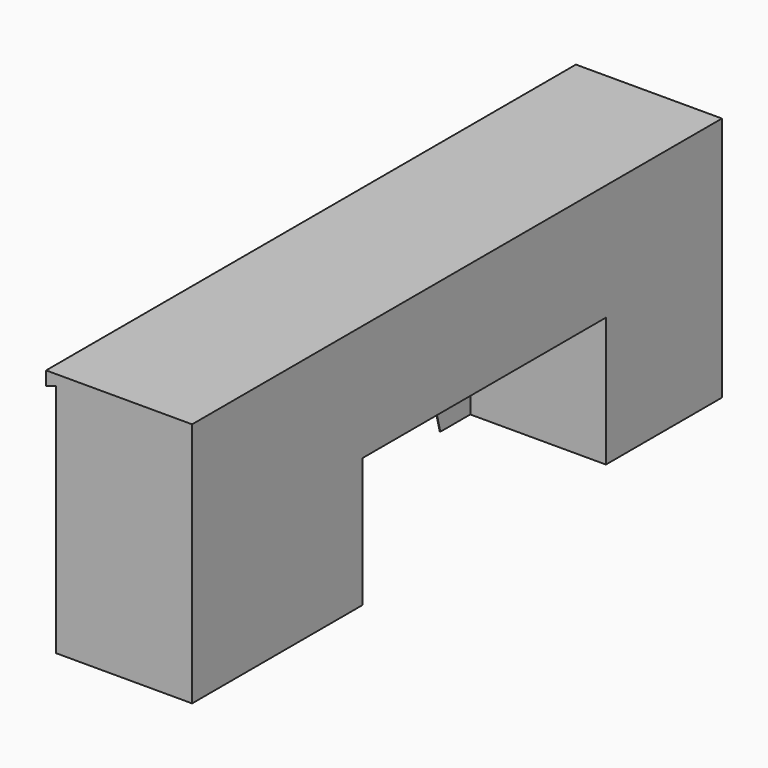
from build123d import *

# Parameters (mm, degrees)
F0_W      = 508
F0_H      = 914.4
F1_DEPTH  = 2470.15
F2_W      = 450.85
F2_H      = 787.4
F2_W_2    = 1060.45
F2_H_2    = 304.8
F2_W_3    = 704.85
F3_DEPTH  = 505.8918
F4_W      = 503.7836
F4_H      = 704.85
F5_DEPTH  = 48.6918
F6_W      = 503.7836
F6_H      = 704.85
F7_DEPTH  = 48.6918
F8_W      = 503.7836
F8_H      = 884.7836
F9_DEPTH  = 37.0459
F10_W     = 503.7836
F10_H     = 884.7836
F11_DEPTH = 48.6918
F12_W     = 503.7836
F12_H     = 1060.45
F13_DEPTH = 48.6918
F14_W     = 503.7836
F14_H     = 1060.45
F15_DEPTH = 48.6918
F16_W     = 503.7836
F16_H     = 402.1836
F17_DEPTH = 37.0459
F18_W     = 503.7836
F18_H     = 402.1836
F19_DEPTH = 37.0459
F20_W     = 503.7836
F20_H     = 450.85
F21_DEPTH = 48.6918
F22_W     = 503.7836
F22_H     = 450.85
F23_DEPTH = 48.6918
F24_W     = 503.7836
F24_H     = 884.7836
F25_DEPTH = 37.0459
F26_W     = 503.7836
F26_H     = 884.7836
F27_DEPTH = 48.6918
F28_W     = 505.8918
F28_H     = 1134.5418
F29_DEPTH = 482.6
F31_DEPTH = 508.001
F33_DEPTH = 2470.15
F34_R     = 0.508
F35_R     = 3.175
F36_DEPTH = 2.1082
F37_R     = 6.35
F38_DEPTH = 2.1082
F39_R     = 6.35
F40_DEPTH = 2.1082


# Not quite as in the source:
# - a feature names something its author has since deleted; it is built from what else it names


with BuildPart() as f1:
    # F0 (on Front) → F1 (new body)
    with BuildSketch(Plane.XZ):
        Rectangle(F0_W, F0_H)
    extrude(amount=-F1_DEPTH)

    # F2 (on face) → F3 (cut)
    with BuildSketch(Plane(origin=(-254, 0, 0), x_dir=(0, -1, 0), z_dir=(-1, 0, 0))):
        with Locations((-2193.925, -12.7)):
            Rectangle(F2_W, F2_H)
        with Locations((-1362.075, 228.6)):
            Rectangle(F2_W_2, F2_H_2)
        with Locations((-403.225, -12.7)):
            Rectangle(F2_W_3, F2_H)
    extrude(amount=-F3_DEPTH, mode=Mode.SUBTRACT)

    # F4 (on face) → F5 (cut)
    with BuildSketch(Plane.XY.offset(-406.4)):
        with Locations((0, 403.225)):
            Rectangle(F4_W, F4_H)
    extrude(amount=-F5_DEPTH, mode=Mode.SUBTRACT)

    # F6 (on face) → F7 (cut)
    with BuildSketch(Plane(origin=(0, 0, 381), x_dir=(1, 0, 0), z_dir=(0, 0, -1))):
        with Locations((0, -403.225)):
            Rectangle(F6_W, F6_H)
    extrude(amount=-F7_DEPTH, mode=Mode.SUBTRACT)

    # F8 (on face) → F9 (cut)
    with BuildSketch(Plane.XZ.offset(-755.65)):
        with Locations((0, -12.7)):
            Rectangle(F8_W, F8_H)
    extrude(amount=-F9_DEPTH, mode=Mode.SUBTRACT)

    # F10 (on face) → F11 (cut)
    with BuildSketch(Plane(origin=(0, 50.8, 0), x_dir=(-1, 0, 0), z_dir=(0, 1, 0))):
        with Locations((0, -12.7)):
            Rectangle(F10_W, F10_H)
    extrude(amount=-F11_DEPTH, mode=Mode.SUBTRACT)

    # F12 (on face) → F13 (cut)
    with BuildSketch(Plane.XY.offset(76.2)):
        with Locations((0, 1362.075)):
            Rectangle(F12_W, F12_H)
    extrude(amount=-F13_DEPTH, mode=Mode.SUBTRACT)

    # F14 (on face) → F15 (cut)
    with BuildSketch(Plane(origin=(0, 0, 381), x_dir=(1, 0, 0), z_dir=(0, 0, -1))):
        with Locations((0, -1362.075)):
            Rectangle(F14_W, F14_H)
    extrude(amount=-F15_DEPTH, mode=Mode.SUBTRACT)

    # F16 (on face) → F17 (cut)
    with BuildSketch(Plane(origin=(0, 831.85, 0), x_dir=(-1, 0, 0), z_dir=(0, 1, 0))):
        with Locations((0, 228.6)):
            Rectangle(F16_W, F16_H)
    extrude(amount=-F17_DEPTH, mode=Mode.SUBTRACT)

    # F18 (on face) → F19 (cut)
    with BuildSketch(Plane.XZ.offset(-1892.3)):
        with Locations((0, 228.6)):
            Rectangle(F18_W, F18_H)
    extrude(amount=-F19_DEPTH, mode=Mode.SUBTRACT)

    # F20 (on face) → F21 (cut)
    with BuildSketch(Plane.XY.offset(-406.4)):
        with Locations((0, 2193.925)):
            Rectangle(F20_W, F20_H)
    extrude(amount=-F21_DEPTH, mode=Mode.SUBTRACT)

    # F22 (on face) → F23 (cut)
    with BuildSketch(Plane(origin=(0, 0, 381), x_dir=(1, 0, 0), z_dir=(0, 0, -1))):
        with Locations((0, -2193.925)):
            Rectangle(F22_W, F22_H)
    extrude(amount=-F23_DEPTH, mode=Mode.SUBTRACT)

    # F24 (on face) → F25 (cut)
    with BuildSketch(Plane(origin=(0, 1968.5, 0), x_dir=(-1, 0, 0), z_dir=(0, 1, 0))):
        with Locations((0, -12.7)):
            Rectangle(F24_W, F24_H)
    extrude(amount=-F25_DEPTH, mode=Mode.SUBTRACT)

    # F26 (on face) → F27 (cut)
    with BuildSketch(Plane.XZ.offset(-2419.35)):
        with Locations((0, -12.7)):
            Rectangle(F26_W, F26_H)
    extrude(amount=-F27_DEPTH, mode=Mode.SUBTRACT)

    # F28 (on face) → F29 (cut)
    with BuildSketch(Plane(origin=(0, 0, -457.2), x_dir=(1, 0, 0), z_dir=(0, 0, -1))):
        with Locations((1.0541, -1362.075)):
            Rectangle(F28_W, F28_H)
    extrude(amount=-F29_DEPTH, mode=Mode.SUBTRACT)

    # F30 (on face) → F31 (cut, through all)
    with BuildSketch(Plane(origin=(-254, 0, 0), x_dir=(0, -1, 0), z_dir=(-1, 0, 0))):
        with BuildLine():
            Line((-1789.6459, -457.2), (-896.4041, -457.2))
            ThreePointArc((-896.4041, -457.2), (-1343.025, -86.7918), (-1789.6459, -457.2))
        make_face()
    extrude(amount=-F31_DEPTH, mode=Mode.SUBTRACT)

    # F32 (on face) → F33 (join, through all)
    with BuildSketch(Plane.XZ):
        Polygon((-290.5981389248, 459.3082), (-290.5981389248, 408.5082), (-254, 419.1), (-254, 457.2), (254, 457.2), (254, 459.3082), align=None)
    extrude(amount=-F33_DEPTH)

    # F34
    f34_edges = [f1.edges().sort_by_distance(p)[0] for p in [
        (-290.598139, 1235.075, 408.5082),
    ]]
    fillet(f34_edges, radius=F34_R)

    # F35 (on face) → F36 (cut, through all)
    with BuildSketch(Plane(origin=(-254, 0, 0), x_dir=(0, -1, 0), z_dir=(-1, 0, 0))):
        with Locations((-1911.35, 38.1)):
            Circle(F35_R)
        with Locations((-812.8, 38.1)):
            Circle(F35_R)
    extrude(amount=-F36_DEPTH, mode=Mode.SUBTRACT)

    # F37 (on face) → F38 (cut, through all)
    with BuildSketch(Plane(origin=(-254, 0, 0), x_dir=(0, -1, 0), z_dir=(-1, 0, 0))):
        with Locations((-29.21, 387.35)):
            Circle(F37_R)
        with Locations((-29.21, -412.75)):
            Circle(F37_R)
    extrude(amount=-F38_DEPTH, mode=Mode.SUBTRACT)

    # F39 (on face) → F40 (cut, through all)
    with BuildSketch(Plane(origin=(-254, 0, 0), x_dir=(0, -1, 0), z_dir=(-1, 0, 0))):
        with Locations((-1946.91, 387.35)):
            Circle(F39_R)
        with Locations((-1946.91, -412.75)):
            Circle(F39_R)
    extrude(amount=-F40_DEPTH, mode=Mode.SUBTRACT)


solid = f1.part
